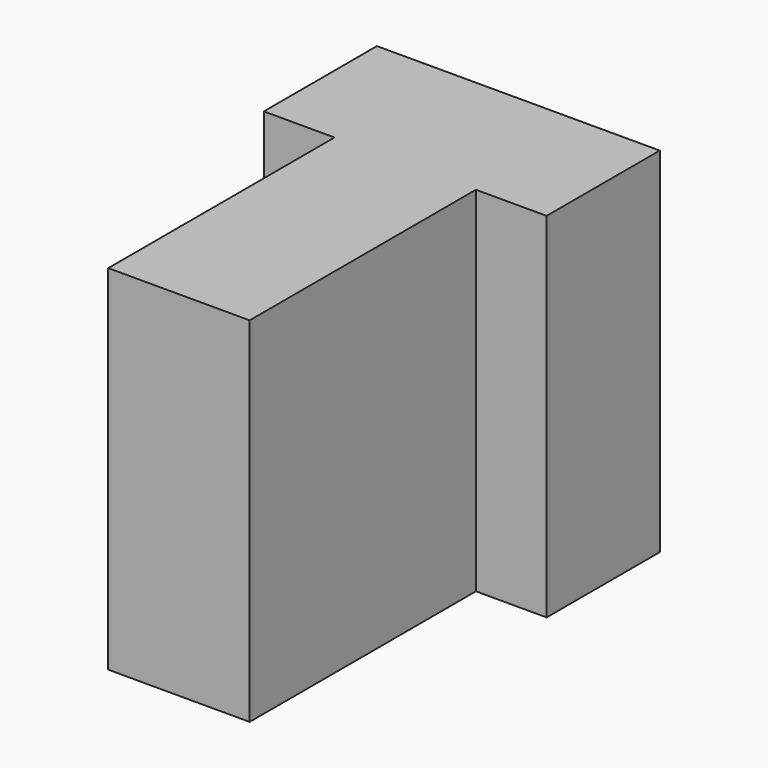
from build123d import *

# Parameters (mm, degrees)
F1_DEPTH = 31.75


# Not quite as in the source:
# - a length typed as a fraction of an inch, garbled in the dataset ("3 / 203.2 mm" for 3/8 in), is restored


with BuildPart() as f1:
    # F0 (on Top) → F1 (new body)
    with BuildSketch(Plane.XY):
        Polygon((-6.35, 25.4), (-6.35, 0), (6.35, 0), (6.35, 25.4), (12.7, 25.4), (12.7, 38.1), (0, 38.1), (-12.7, 38.1), (-12.7, 25.4), align=None)
    extrude(amount=F1_DEPTH)


solid = f1.part
